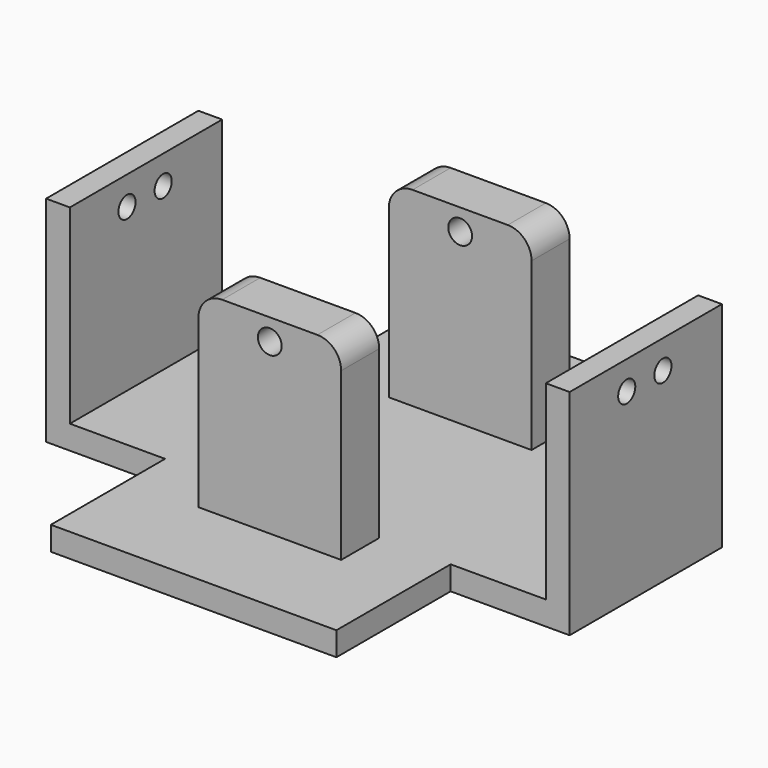
from build123d import *

# Parameters (mm, degrees)
F0_W      = 30
F0_H      = 100
F1_DEPTH  = 5
F2_W      = 30
F2_H      = 10
F3_DEPTH  = 40
F4_R      = 5
F5_R      = 2.5
F6_DEPTH  = 80.001
F7_W      = 40
F7_H      = 5
F8_DEPTH  = 25
F9_W      = 5
F9_H      = 40
F10_DEPTH = 40
F11_R     = 2.25
F12_DEPTH = 25


with BuildPart() as f1:
    # F0 (on Top) → F1 (new body)
    with BuildSketch(Plane.XY):
        with Locations((-15, 0)):
            Rectangle(F0_W, F0_H)
        with Locations((15, 0)):
            Rectangle(F0_W, F0_H)
    extrude(amount=F1_DEPTH)

    # F2 (on face) → F3 (join)
    with BuildSketch(Plane.XY.offset(5)):
        with Locations((0, 25)):
            Rectangle(F2_W, F2_H)
        with Locations((0, -25)):
            Rectangle(F2_W, F2_H)
    extrude(amount=F3_DEPTH)

    # F4
    f4_edges = [f1.edges().sort_by_distance(p)[0] for p in [
        (-15, -25, 45),
        (15, -25, 45),
        (-15, 25, 45),
        (15, 25, 45),
    ]]
    fillet(f4_edges, radius=F4_R)

    # F5 (on face) → F6 (cut, through all)
    with BuildSketch(Plane.XZ.offset(30)):
        with Locations((0, 40.5)):
            Circle(F5_R)
    extrude(amount=-F6_DEPTH, mode=Mode.SUBTRACT)

    # F7 (on face) → F8 (join)
    with BuildSketch(Plane.YZ.offset(30)):
        with Locations((0, 2.5)):
            Rectangle(F7_W, F7_H)
    extrude(amount=F8_DEPTH)

    # F9 (on face) → F10 (join)
    with BuildSketch(Plane.XY.offset(5)):
        with Locations((52.5, 0)):
            Rectangle(F9_W, F9_H)
    extrude(amount=F10_DEPTH)

    # F11 (on face) → F12 (cut)
    with BuildSketch(Plane.YZ.offset(55)):
        with Locations((-5, 39)):
            Circle(F11_R)
        with Locations((4.5, 39)):
            Circle(F11_R)
    extrude(amount=-F12_DEPTH, mode=Mode.SUBTRACT)

    # F15: F1 across plane


with BuildPart() as f1_1:
    add(f1.part)
    add(f1.part.mirror(Plane(origin=(0, 0, 5.5), x_dir=(0, -1, 0), z_dir=(-1, 0, 0))))


solid = f1_1.part
